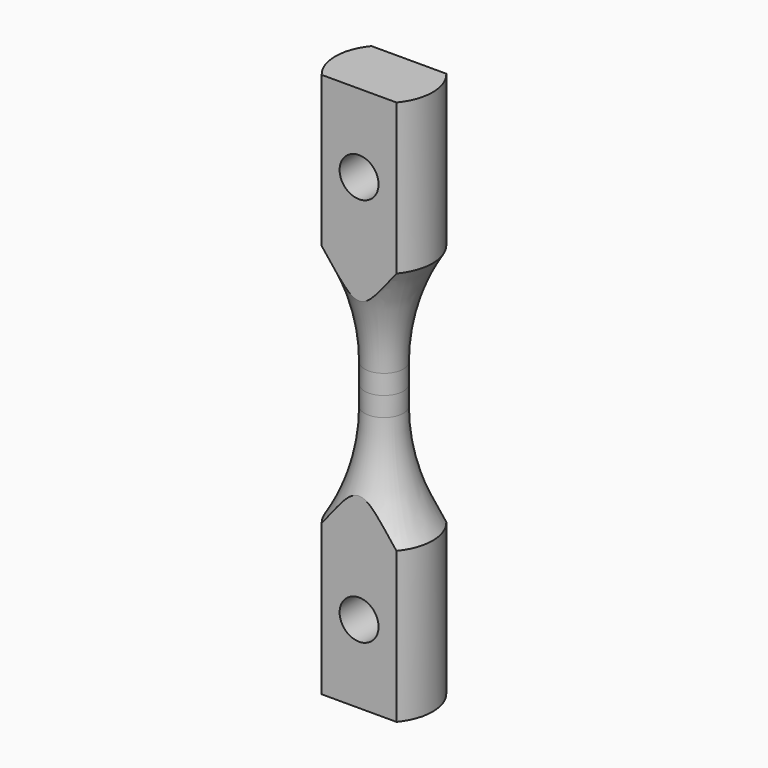
from build123d import *

# Parameters (mm, degrees)
F2_W     = 1.25
F2_H     = 7
F3_DEPTH = 0.8
F4_R     = 0.5
F5_DEPTH = 12.5


# Not quite as in the source:
# - a feature names something its author has since deleted; it is built from what else it names


with BuildPart() as f1:
    # F0 (on Front) → F1 (revolve)
    with BuildSketch(Plane.XZ):
        with BuildLine():
            Line((1.25, 7), (0, 7))
            Line((0, 7), (0, 0))
            Line((0, 0), (0, -7))
            Line((0, -7), (1.25, -7))
            Line((1.25, -7), (1.25, -3.1339134382))
            ThreePointArc((1.25, -3.1339134382), (0.6911539846, -1.8693063938), (0.5, -0.5))
            Line((0.5, -0.5), (0.5, 0.5))
            ThreePointArc((0.5, 0.5), (0.6911539846, 1.8693063938), (1.25, 3.1339134382))
            Line((1.25, 3.1339134382), (1.25, 7))
        make_face()
    revolve(axis=Axis((0, 0, 3.5), (0, 0, -1)))

    # F2 (on Front) → F3 (intersect, symmetric)
    with BuildSketch(Plane.XZ):
        with Locations((0.625, 3.5)):
            Rectangle(F2_W, F2_H)
        with Locations((-0.625, 3.5)):
            Rectangle(F2_W, F2_H)
    extrude(amount=F3_DEPTH, both=True, mode=Mode.INTERSECT)

    # F4 (on Front) → F5 (cut, symmetric)
    with BuildSketch(Plane.XZ):
        with Locations((0, 5)):
            Circle(F4_R)
    extrude(amount=F5_DEPTH, both=True, mode=Mode.SUBTRACT)

    # F6: F1 across plane


with BuildPart() as f1_1:
    add(f1.part)
    add(f1.part.mirror(Plane.XY))


solid = f1_1.part
